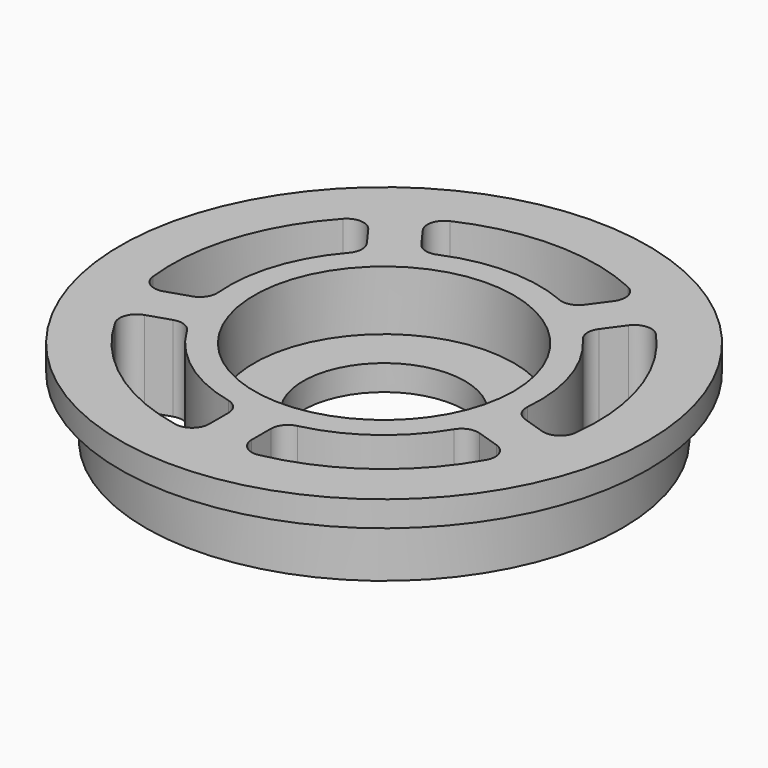
from build123d import *

# Parameters (mm, degrees)
F0_R     = 15.25
F0_R_2   = 9.5
F1_DEPTH = 3
F0_R_3   = 28
F2_DEPTH = 10
F3_R     = 31
F3_R_2   = 28
F4_DEPTH = 3
F5_R     = 2


# Not quite as in the source:
# - a feature names something its author has since deleted; it is built from what else it names


with BuildPart() as f1:
    # F0 (on Top) → F1 (new body)
    with BuildSketch(Plane.XY):
        with Locations((-39.1464792192, 0)):
            Circle(F0_R)
        with Locations((-39.1464792192, 0)):
            Circle(F0_R_2, mode=Mode.SUBTRACT)
    extrude(amount=F1_DEPTH)


with BuildPart() as f2:
    # F0 (on Top) → F2 (new body)
    with BuildSketch(Plane.XY):
        with Locations((-39.1464792192, 0)):
            Circle(F0_R_3)
        with BuildLine():
            ThreePointArc((-41.6464792192, -24.8746859277), (-53.8411105265, -20.2254248594), (-62.0311688756, -10.0643419721))
            Line((-62.0311688756, -10.0643419721), (-55.5670947689, -7.9640369769))
            ThreePointArc((-55.5670947689, -7.9640369769), (-49.8735600735, -14.7645601473), (-41.6464792192, -18.0779561898))
            Line((-41.6464792192, -18.0779561898), (-41.6464792192, -24.8746859277))
        make_face(mode=Mode.SUBTRACT)
        with BuildLine():
            Line((-36.6464792192, -24.8746859277), (-36.6464792192, -18.0779561898))
            ThreePointArc((-36.6464792192, -18.0779561898), (-28.4193983649, -14.7645601473), (-22.7258636695, -7.9640369769))
            Line((-22.7258636695, -7.9640369769), (-16.2617895628, -10.0643419721))
            ThreePointArc((-16.2617895628, -10.0643419721), (-24.4518479119, -20.2254248594), (-36.6464792192, -24.8746859277))
        make_face(mode=Mode.SUBTRACT)
        with BuildLine():
            ThreePointArc((-51.7949777451, 13.1559106504), (-56.5032606416, 5.6395601473), (-57.1121797407, -3.2087543955))
            Line((-57.1121797407, -3.2087543955), (-63.5762538474, -5.3090593907))
            ThreePointArc((-63.5762538474, -5.3090593907), (-62.9228921266, 7.7254248594), (-55.7899952488, 18.6545805145))
            Line((-55.7899952488, 18.6545805145), (-51.7949777451, 13.1559106504))
        make_face(mode=Mode.SUBTRACT)
        with BuildLine():
            ThreePointArc((-30.5430656652, 16.0948369118), (-39.1464792192, 18.25), (-47.7498927732, 16.0948369118))
            Line((-47.7498927732, 16.0948369118), (-51.7449102769, 21.593506776))
            ThreePointArc((-51.7449102769, 21.593506776), (-39.1464792192, 25), (-26.5480481614, 21.593506776))
            Line((-26.5480481614, 21.593506776), (-30.5430656652, 16.0948369118))
        make_face(mode=Mode.SUBTRACT)
        with Locations((-39.1464792192, 0)):
            Circle(F0_R, mode=Mode.SUBTRACT)
        with BuildLine():
            ThreePointArc((-21.1807786977, -3.2087543955), (-21.7896977968, 5.6395601473), (-26.4979806933, 13.1559106504))
            Line((-26.4979806933, 13.1559106504), (-22.5029631896, 18.6545805145))
            ThreePointArc((-22.5029631896, 18.6545805145), (-15.3700663118, 7.7254248594), (-14.716704591, -5.3090593907))
            Line((-14.716704591, -5.3090593907), (-21.1807786977, -3.2087543955))
        make_face(mode=Mode.SUBTRACT)
    extrude(amount=F2_DEPTH)

    # F3 (on face) → F4 (join)
    with BuildSketch(Plane.XY.offset(10)):
        with Locations((-39.1464792192, 0)):
            Circle(F3_R)
        with Locations((-39.1464792192, 0)):
            Circle(F3_R_2, mode=Mode.SUBTRACT)
    extrude(amount=-F4_DEPTH)

    # F5
    f5_edges = [f2.edges().sort_by_distance(p)[0] for p in [
        (-62.031169, -10.064342, 5),
        (-55.567095, -7.964037, 5),
        (-41.646479, -24.874686, 5),
        (-41.646479, -18.077956, 5),
        (-36.646479, -18.077956, 5),
        (-36.646479, -24.874686, 5),
        (-16.26179, -10.064342, 5),
        (-22.725864, -7.964037, 5),
        (-14.716705, -5.309059, 5),
        (-21.180779, -3.208754, 5),
        (-26.497981, 13.155911, 5),
        (-22.502963, 18.654581, 5),
        (-26.548048, 21.593507, 5),
        (-30.543066, 16.094837, 5),
        (-47.749893, 16.094837, 5),
        (-51.74491, 21.593507, 5),
        (-51.794978, 13.155911, 5),
        (-57.11218, -3.208754, 5),
        (-63.576254, -5.309059, 5),
        (-55.789995, 18.654581, 5),
    ]]
    fillet(f5_edges, radius=F5_R)


solid = Compound([f1.part, f2.part])
